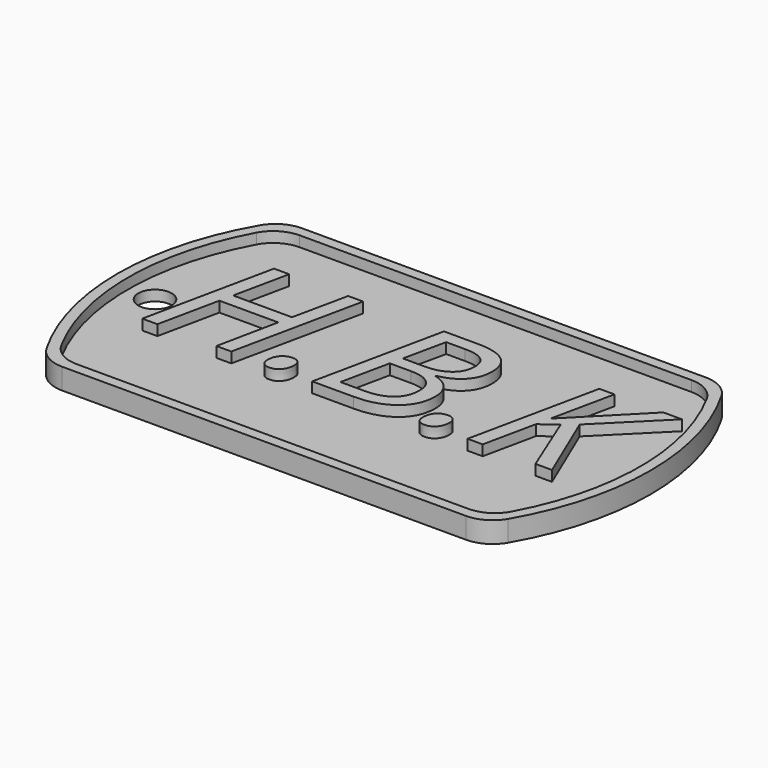
from build123d import *

# Parameters (mm, degrees)
F1_DEPTH     = 1
F3_DEPTH     = 1
F4_R         = 1.5875
F5_DEPTH     = 1
F6_TEXT_SIZE = 17.3904544984
F7_DEPTH     = 1


# Not quite as in the source:
# - Text() gives the source's letters only with a copy of the font that has no kerning and outlines rounded to 1/6400 em; it was checked with that copy


with BuildPart() as f1:
    # F0 (on Top) → F1 (new body)
    with BuildSketch(Plane.XY):
        with BuildLine():
            ThreePointArc((-19.2474145991, 14.2875), (-20.8349145991, 13.862130657), (-21.9970452561, 12.7))
            ThreePointArc((-21.9970452561, 12.7), (-25.4, 0), (-21.9970452561, -12.7))
            ThreePointArc((-21.9970452561, -12.7), (-20.8349145991, -13.862130657), (-19.2474145991, -14.2875))
            Line((-19.2474145991, -14.2875), (19.2474145991, -14.2875))
            ThreePointArc((19.2474145991, -14.2875), (20.8349145991, -13.862130657), (21.9970452561, -12.7))
            ThreePointArc((21.9970452561, -12.7), (25.4, 0), (21.9970452561, 12.7))
            ThreePointArc((21.9970452561, 12.7), (20.8349145991, 13.862130657), (19.2474145991, 14.2875))
            Line((19.2474145991, 14.2875), (-19.2474145991, 14.2875))
        make_face()
    extrude(amount=F1_DEPTH)

    # F2 (on face) → F3 (join)
    with BuildSketch(Plane.XY.offset(1)):
        with BuildLine():
            Line((19.2474145991, 14.2875), (-19.2474145991, 14.2875))
            ThreePointArc((-19.2474145991, 14.2875), (-20.8349145991, 13.862130657), (-21.9970452561, 12.7))
            ThreePointArc((-21.9970452561, 12.7), (-25.4, 0), (-21.9970452561, -12.7))
            ThreePointArc((-21.9970452561, -12.7), (-20.8349145991, -13.862130657), (-19.2474145991, -14.2875))
            Line((-19.2474145991, -14.2875), (19.2474145991, -14.2875))
            ThreePointArc((19.2474145991, -14.2875), (20.8349145991, -13.862130657), (21.9970452561, -12.7))
            ThreePointArc((21.9970452561, -12.7), (25.4, 0), (21.9970452561, 12.7))
            ThreePointArc((21.9970452561, 12.7), (20.8349145991, 13.862130657), (19.2474145991, 14.2875))
        make_face()
        with BuildLine():
            ThreePointArc((-21.4526124879, 11.6252061249), (-20.2856017842, 12.8404540819), (-18.6611352482, 13.2875))
            Line((-18.6611352482, 13.2875), (18.6611352482, 13.2875))
            ThreePointArc((18.6611352482, 13.2875), (20.2856017842, 12.8404540819), (21.4526124879, 11.6252061249))
            ThreePointArc((21.4526124879, 11.6252061249), (24.4, 0), (21.4526124879, -11.6252061249))
            ThreePointArc((21.4526124879, -11.6252061249), (20.2856017842, -12.8404540819), (18.6611352482, -13.2875))
            Line((18.6611352482, -13.2875), (-18.6611352482, -13.2875))
            ThreePointArc((-18.6611352482, -13.2875), (-20.2856017842, -12.8404540819), (-21.4526124879, -11.6252061249))
            ThreePointArc((-21.4526124879, -11.6252061249), (-24.4, 0), (-21.4526124879, 11.6252061249))
        make_face(mode=Mode.SUBTRACT)
    extrude(amount=F3_DEPTH)

    # F4 (on face) → F5 (cut)
    with BuildSketch(Plane.XY.offset(1)):
        with Locations((-21.821282804, 0)):
            Circle(F4_R)
    extrude(amount=-F5_DEPTH, mode=Mode.SUBTRACT)

    # F6 (on face) → F7 (join)
    with BuildSketch(Plane.XY.offset(1)):
        with Locations((-20.1590147335, -4.5076054521)):
            Text('H.B.K', F6_TEXT_SIZE, font='Open Sans', font_style=FontStyle.ITALIC, text_align=(TextAlign.LEFT, TextAlign.BOTTOM))
    extrude(amount=F7_DEPTH)


solid = f1.part
